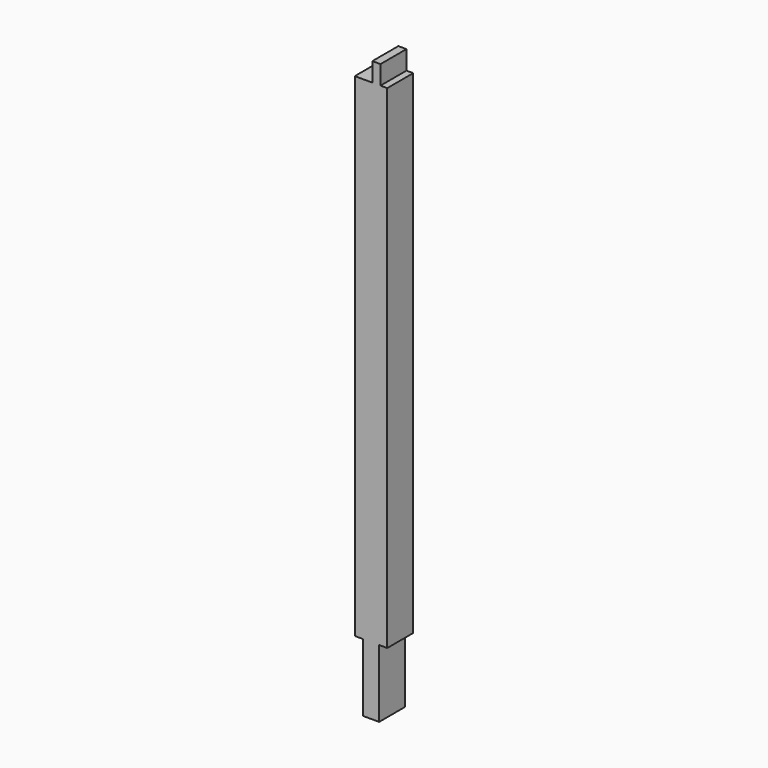
from build123d import *

# Parameters (mm, degrees)
F0_W     = 38.1
F0_H     = 88.9
F1_DEPTH = 76.2
F2_W     = 76.2
F2_H     = 152.4
F3_DEPTH = 317.5


# Not quite as in the source:
# - a feature names something its author has since deleted; it is built from what else it names


with BuildPart() as f1:
    # F0 (on Front) → F1 (new body, symmetric)
    with BuildSketch(Plane.XZ):
        Polygon((6.35, 1111.25), (-76.2, 1111.25), (-76.2, -1200.15), (76.2, -1200.15), (76.2, 1111.25), (44.45, 1111.25), align=None)
        with Locations((25.4, 1155.7)):
            Rectangle(F0_W, F0_H)
    extrude(amount=F1_DEPTH, both=True)

    # F2 (on face) → F3 (join)
    with BuildSketch(Plane(origin=(0, 0, -1200.15), x_dir=(1, 0, 0), z_dir=(0, 0, -1))):
        Rectangle(F2_W, F2_H)
    extrude(amount=F3_DEPTH)


solid = f1.part
